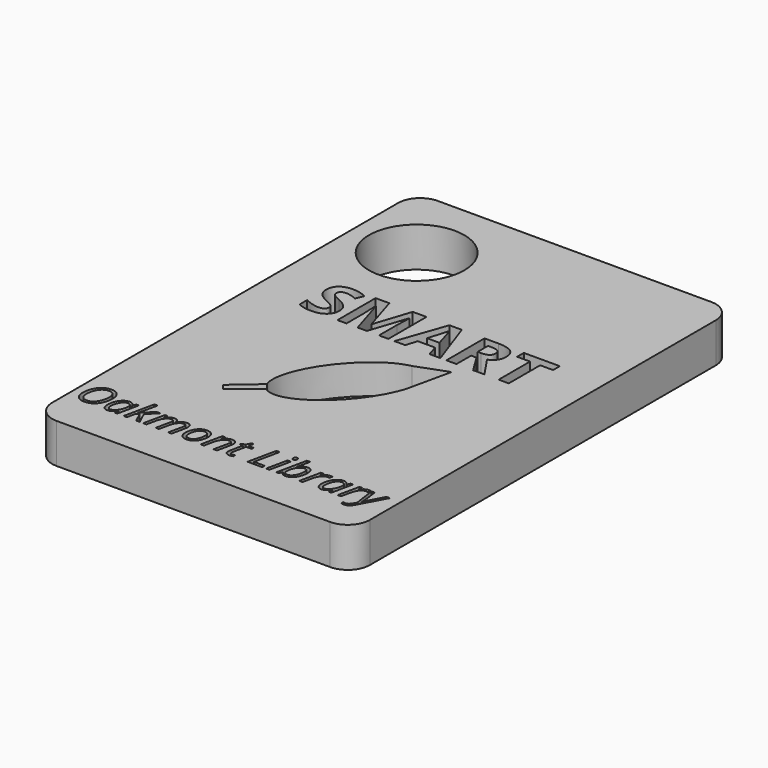
from build123d import *

# Parameters (mm, degrees)
F0_W         = 20.32
F0_H         = 30.48
F1_DEPTH     = 2.54
F2_TEXT_SIZE = 4.2664249324
F3_DEPTH     = 1.905
F4_R         = 1.4103835631
F5_TEXT_SIZE = 2.5604736505
F6_DEPTH     = 1.905
F7_R         = 3.048
F8_DEPTH     = 25.4
F10_DEPTH    = 1.905


# Not quite as in the source:
# - Text() gives the source's letters only with a copy of the font that has no kerning and outlines rounded to 1/6400 em; it was checked with that copy


with BuildPart() as f1:
    # F0 (on Top) → F1 (new body)
    with BuildSketch(Plane.XY):
        Rectangle(F0_W, F0_H)
    extrude(amount=F1_DEPTH)

    # F2 (on face) → F3 (cut)
    with BuildSketch(Plane.XY.offset(2.54)):
        with Locations((-7.3422436835, 2.0414288156)):
            Text('SMART', F2_TEXT_SIZE, font='Open Sans', font_style=FontStyle.BOLD, text_align=(TextAlign.LEFT, TextAlign.BOTTOM))
    extrude(amount=-F3_DEPTH, mode=Mode.SUBTRACT)

    # F4
    f4_edges = [f1.edges().sort_by_distance(p)[0] for p in [
        (-10.16, 15.24, 1.27),
        (10.16, 15.24, 1.27),
        (10.16, -15.24, 1.27),
        (-10.16, -15.24, 1.27),
    ]]
    fillet(f4_edges, radius=F4_R)

    # F5 (on face) → F6 (cut)
    with BuildSketch(Plane.XY.offset(2.54)):
        with Locations((-9.8330489336, -12.731081845)):
            Text('Oakmont Library', F5_TEXT_SIZE, font='Open Sans', font_style=FontStyle.ITALIC, text_align=(TextAlign.LEFT, TextAlign.BOTTOM))
    extrude(amount=-F6_DEPTH, mode=Mode.SUBTRACT)

    # F7 (on face) → F8 (cut)
    with BuildSketch(Plane.XY.offset(2.54)):
        with Locations((-6.074977914, 10.2056851854)):
            Circle(F7_R)
    extrude(amount=-F8_DEPTH, mode=Mode.SUBTRACT)

    # F9 (on face) → F10 (cut)
    with BuildSketch(Plane.XY.offset(2.54)):
        with BuildLine():
            add(Edge.make_bspline(
                [(-3.0383281397, -5.5692818653), (-2.9397402609, -5.8266232834), (-2.748648636, -5.9856099542)],
                knots=[6.0255411869, 6.0255411869, 6.0255411869, 6.2831853072, 6.2831853072, 6.2831853072], degree=2, weights=[1, 0.991713907, 1]))
            add(Edge.make_bspline(
                [(-2.748648636, -5.9856099542), (-2.7421998036, -5.9909753301), (-2.7356514048, -5.9962205323)],
                knots=[0, 0, 0, 0.0087431644, 0.0087431644, 0.0087431644], degree=2, weights=[1, 0.9999904446, 1]))
            add(Edge.make_bspline(
                [(-2.7356514048, -5.9962205323), (0.805238379, -8.8324379409), (2.7473773114, -1.5146030064)],
                knots=[0.0087431644, 0.0087431644, 0.0087431644, 2.3499173593, 2.3499173593, 2.3499173593], degree=2, weights=[1, 0.3896110468, 1]))
            Line((2.7473773114, -1.5146030064), (2.8178843574, -1.1958617528))
            add(Edge.make_bspline(
                [(2.8178843574, -1.1958617528), (3.1720978782, 0.8323765496), (1.3902529848, 0.485798349)],
                knots=[2.4554696615, 2.4554696615, 2.4554696615, 3.6638574773, 3.6638574773, 3.6638574773], degree=2, weights=[1, 0.822960305, 1]))
            add(Edge.make_bspline(
                [(1.3902529848, 0.485798349), (-4.8900592908, -0.7357554099), (-3.0383281397, -5.5692818653)],
                knots=[3.6638574773, 3.6638574773, 3.6638574773, 6.0255411869, 6.0255411869, 6.0255411869], degree=2, weights=[1, 0.3801463055, 1]))
        make_face()
        with BuildLine():
            add(Edge.make_bspline(
                [(-2.748648636, -5.9856099542), (-2.7421998036, -5.9909753301), (-2.7356514048, -5.9962205323)],
                knots=[0, 0, 0, 0.0087431644, 0.0087431644, 0.0087431644], degree=2, weights=[1, 0.9999904446, 1]))
            add(Edge.make_bspline(
                [(-3.0383281397, -5.5692818653), (-2.9397402609, -5.8266232834), (-2.748648636, -5.9856099542)],
                knots=[6.0255411869, 6.0255411869, 6.0255411869, 6.2831853072, 6.2831853072, 6.2831853072], degree=2, weights=[1, 0.991713907, 1]))
            Line((-3.0383281397, -5.5692818653), (-4.7055765546, -7.0068757773))
            Line((-4.7055765546, -7.0068757773), (-4.4424813241, -7.3408423923))
            Line((-4.4424813241, -7.3408423923), (-2.7356514048, -5.9962205323))
        make_face()
        with BuildLine():
            Line((2.8178843574, -1.1958617528), (2.7473773114, -1.5146030064))
            add(Edge.make_bspline(
                [(2.7473773114, -1.5146030064), (2.7907786165, -1.3510701196), (2.8178843574, -1.1958617528)],
                knots=[2.3499173593, 2.3499173593, 2.3499173593, 2.4554696615, 2.4554696615, 2.4554696615], degree=2, weights=[1, 0.9986076622, 1]))
        make_face()
        with BuildLine():
            Line((3.3511425072, 1.2148387481), (1.3902529848, 0.485798349))
            add(Edge.make_bspline(
                [(2.8178843574, -1.1958617528), (3.1720978782, 0.8323765496), (1.3902529848, 0.485798349)],
                knots=[2.4554696615, 2.4554696615, 2.4554696615, 3.6638574773, 3.6638574773, 3.6638574773], degree=2, weights=[1, 0.822960305, 1]))
            Line((2.8178843574, -1.1958617528), (3.3511425072, 1.2148387481))
        make_face()
    extrude(amount=-F10_DEPTH, mode=Mode.SUBTRACT)


solid = f1.part
